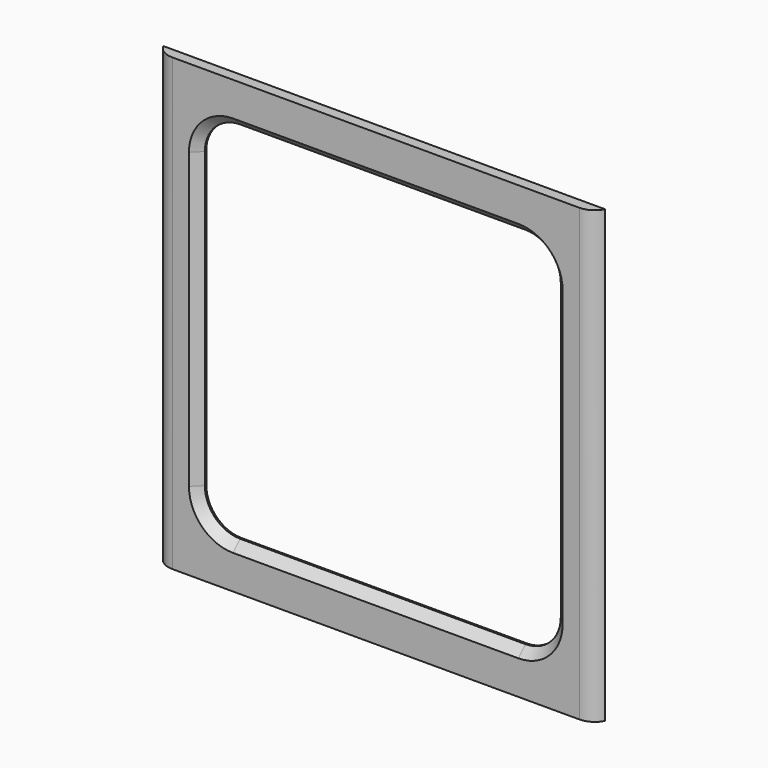
from build123d import *

# Parameters (mm, degrees)
F0_W        = 500
F0_H        = 510
F1_DEPTH    = 12
F2_SIZE     = 10
F3_T1_DEPTH = 607.9795897113


# Not quite as in the source:
# - a fillet or chamfer that OpenCascade refuses, or shapes differently, is made with other operations: its cross-section is extruded or revolved along the edge and cut away or added


with BuildPart() as f1:
    # F0 (on Front) → F1 (new body)
    with BuildSketch(Plane.XZ):
        with Locations((1.5247634146, 0)):
            Rectangle(F0_W, F0_H)
        with BuildLine():
            ThreePointArc((-199.9752365854, 166.5), (-188.2595078328, 194.7842712475), (-159.9752365854, 206.5))
            Line((-159.9752365854, 206.5), (163.0247634146, 206.5))
            ThreePointArc((163.0247634146, 206.5), (191.3090346621, 194.7842712475), (203.0247634146, 166.5))
            Line((203.0247634146, 166.5), (203.0247634146, -166.5))
            ThreePointArc((203.0247634146, -166.5), (191.3090346621, -194.7842712475), (163.0247634146, -206.5))
            Line((163.0247634146, -206.5), (-159.9752365854, -206.5))
            ThreePointArc((-159.9752365854, -206.5), (-188.2595078328, -194.7842712475), (-199.9752365854, -166.5))
            Line((-199.9752365854, -166.5), (-199.9752365854, 166.5))
        make_face(mode=Mode.SUBTRACT)
    extrude(amount=F1_DEPTH)

    # F2
    f2_edges = [f1.edges().sort_by_distance(p)[0] for p in [
        (1.524763, -12, 206.5),
        (-199.975237, -12, 0),
        (-188.259508, -12, 194.784271),
        (191.309035, -12, 194.784271),
        (203.024763, -12, 0),
        (191.309035, -12, -194.784271),
        (1.524763, -12, -206.5),
        (-188.259508, -12, -194.784271),
    ]]
    chamfer(f2_edges, length=F2_SIZE)

    # F3: fillet of radius 22 on 2 edges, made by hand

    # F3_s2 → F3_t1 (cut)
    with BuildSketch(Plane.XY.offset(-303.9897948557)):
        with BuildLine():
            ThreePointArc((-228.8793186431, -12), (-240.3684439362, -8.7616630393), (-248.4752365854, 0))
            Line((-248.4752365854, 0), (-248.4752365854, -12))
            Line((-248.4752365854, -12), (-228.8793186431, -12))
        make_face()
        with BuildLine():
            ThreePointArc((231.9288454724, -12), (243.4179707654, -8.7616630393), (251.5247634146, 0))
            Line((251.5247634146, 0), (251.5247634146, -12))
            Line((251.5247634146, -12), (231.9288454724, -12))
        make_face()
    extrude(amount=F3_T1_DEPTH, mode=Mode.SUBTRACT)


solid = f1.part
